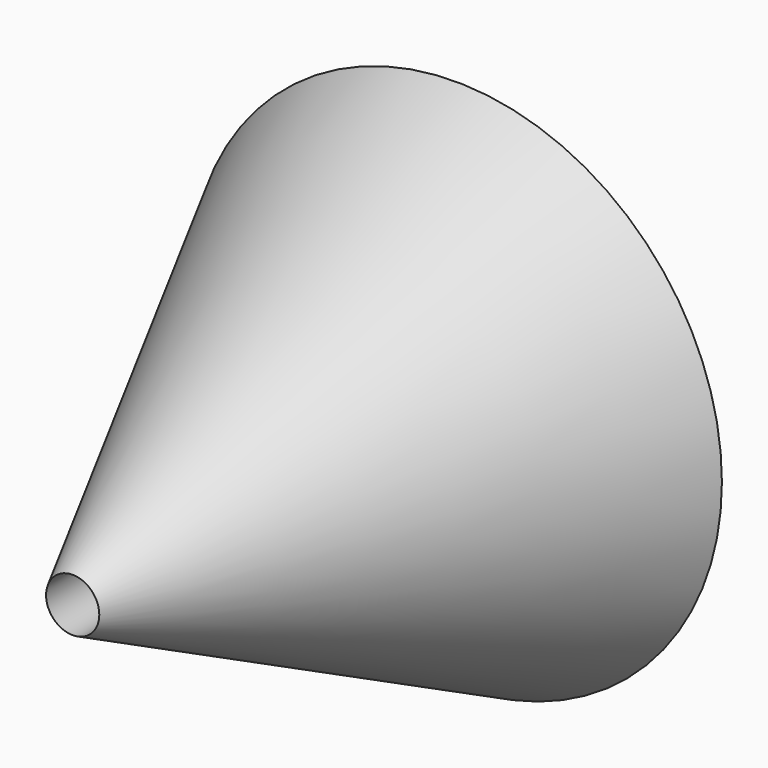
from build123d import *

# Parameters (mm, degrees)
F0_R     = 1.27
F1_DEPTH = 2.54
F2_SIZE2 = 2.53999
F2_SIZE  = 1.26999
F3_R     = 0.127
F4_DEPTH = 2.541


# Not quite as in the source:
# - a fillet or chamfer is up to 0.001 mm smaller than in the source, because OpenCascade refuses the exact size


with BuildPart() as f1:
    # F0 (on Front) → F1 (new body)
    with BuildSketch(Plane.XZ):
        Circle(F0_R)
    extrude(amount=F1_DEPTH)

    # F2 (size 1.27 and 2.54 in the source; OpenCascade refuses exactly that, so slightly less here)
    f2_edges = [f1.edges().sort_by_distance(p)[0] for p in [
        (-1.27, -2.54, 0),
    ]]
    f2_side = f1.faces().sort_by_distance((0, -2.54, 0))[0]
    chamfer(f2_edges, length=F2_SIZE, length2=F2_SIZE2, reference=f2_side)

    # F3 (on face) → F4 (cut, through all)
    with BuildSketch(Plane(origin=(0, 0, 0), x_dir=(-1, 0, 0), z_dir=(0, 1, 0))):
        Circle(F3_R)
    extrude(amount=-F4_DEPTH, mode=Mode.SUBTRACT)


solid = f1.part
